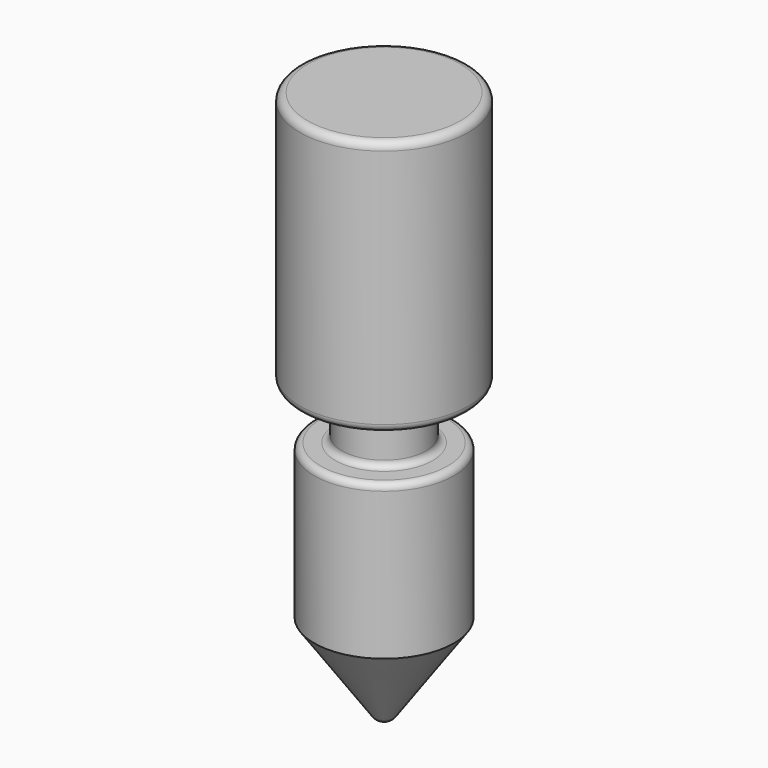
from build123d import *

# Parameters (mm, degrees)
F2_R = 0.3066051224
F3_R = 0.4318
F4_R = 0.254


# Not quite as in the source:
# - a feature names something its author has since deleted; it is built from what else it names


with BuildPart() as f1:
    # F0 (on Front) → F1 (revolve)
    with BuildSketch(Plane.XZ):
        Polygon((3.9006043464, 21.6174807614), (0.5986043464, 21.6174807614), (0.5986043464, 0), (0.8526043464, 0), (3.3346717246, 3.5295289444), (3.3346717246, 9.5524807614), (2.2496043464, 9.5524807614), (2.2496043464, 11.5844807614), (3.9006043464, 11.5844807614), align=None)
    revolve(axis=Axis((0.5986043464, 0, 10.8087403807), (0, 0, -1)))

    # F2
    f2_edges = [f1.edges().sort_by_distance(p)[0] for p in [
        (-2.703396, 0, 21.617481),
        (-2.703396, 0, 11.584481),
    ]]
    fillet(f2_edges, radius=F2_R)

    # F3
    f3_edges = [f1.edges().sort_by_distance(p)[0] for p in [
        (0.344604, 0, 0),
    ]]
    fillet(f3_edges, radius=F3_R)

    # F4
    f4_edges = [f1.edges().sort_by_distance(p)[0] for p in [
        (-2.137463, 0, 9.552481),
        (-1.052396, 0, 9.552481),
    ]]
    fillet(f4_edges, radius=F4_R)


solid = f1.part
